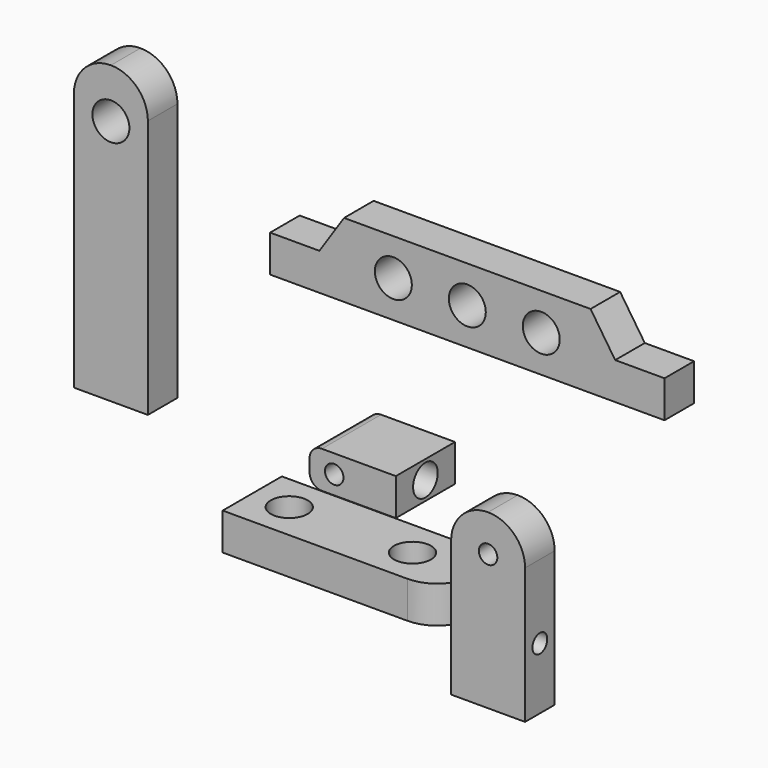
from build123d import *

# Parameters (mm, degrees)
F0_W      = 44.45
F0_H      = 19.05
F1_DEPTH  = 38.1
F2_R      = 4.7625
F3_DEPTH  = 118.58277
F4_R      = 7.9375
F5_DEPTH  = 12.7
F6_R      = 6.35
F7_W      = 38.1
F7_H      = 88.9
F7_R      = 4.7625
F8_DEPTH  = 19.05
F9_R      = 4.7625
F10_DEPTH = 19.05
F11_R     = 19.04999
F12_W     = 114.3
F12_H     = 19.05
F13_DEPTH = 38.1
F14_R     = 9.525
F15_DEPTH = 43.37852
F16_R     = 19.04999
F17_R     = 9.525
F18_DEPTH = 19.05
F19_R     = 9.525
F20_DEPTH = 19.05


# Not quite as in the source:
# - a fillet or chamfer is up to 0.001 mm smaller than in the source, because OpenCascade refuses the exact size


with BuildPart() as f1:
    # F0 (on Front) → F1 (new body)
    with BuildSketch(Plane.XZ):
        with Locations((-4.5246369214, 25.4022409208)):
            Rectangle(F0_W, F0_H)
    extrude(amount=-F1_DEPTH)

    # F2 (on face) → F3 (cut)
    with BuildSketch(Plane.XZ):
        with Locations((-14.0496369214, 25.4022409208)):
            Circle(F2_R)
    extrude(amount=-F3_DEPTH, mode=Mode.SUBTRACT)

    # F4 (on face) → F5 (cut)
    with BuildSketch(Plane.YZ.offset(17.7003630786)):
        with Locations((19.05, 25.4022409208)):
            Circle(F4_R)
    extrude(amount=-F5_DEPTH, mode=Mode.SUBTRACT)

    # F6
    f6_edges = [f1.edges().sort_by_distance(p)[0] for p in [
        (-26.749637, 19.05, 34.927241),
        (-26.749637, 19.05, 15.877241),
    ]]
    fillet(f6_edges, radius=F6_R)


with BuildPart() as f8:
    # F7 (on Front) → F8 (new body)
    with BuildSketch(Plane.XZ):
        with Locations((65.2318205684, -10.4596508645)):
            Rectangle(F7_W, F7_H)
        with Locations((65.2318205684, 14.9403491355)):
            Circle(F7_R, mode=Mode.SUBTRACT)
    extrude(amount=-F8_DEPTH)

    # F9 (on face) → F10 (cut)
    with BuildSketch(Plane.YZ.offset(84.2818205684)):
        with Locations((9.525, -23.1596508645)):
            Circle(F9_R)
    extrude(amount=-F10_DEPTH, mode=Mode.SUBTRACT)

    # F11 (radius 19.05 in the source; OpenCascade refuses exactly that, so slightly less here)
    f11_edges = [f8.edges().sort_by_distance(p)[0] for p in [
        (84.281821, 9.525, 33.990349),
        (46.181821, 9.525, 33.990349),
    ]]
    fillet(f11_edges, radius=F11_R)


with BuildPart() as f13:
    # F12 (on Front) → F13 (new body)
    with BuildSketch(Plane.XZ):
        with Locations((-14.3527926165, -19.2319881171)):
            Rectangle(F12_W, F12_H)
    extrude(amount=-F13_DEPTH)

    # F14 (on face) → F15 (cut)
    with BuildSketch(Plane.XY.offset(-9.7069881171)):
        with Locations((-52.4527926165, 19.05)):
            Circle(F14_R)
        with Locations((11.0472073835, 19.05)):
            Circle(F14_R)
    extrude(amount=-F15_DEPTH, mode=Mode.SUBTRACT)

    # F16 (radius 19.05 in the source; OpenCascade refuses exactly that, so slightly less here)
    f16_edges = [f13.edges().sort_by_distance(p)[0] for p in [
        (42.797207, 38.1, -19.231988),
        (42.797207, 0, -19.231988),
    ]]
    fillet(f16_edges, radius=F16_R)


with BuildPart() as f18:
    # F17 (on Front) → F18 (new body)
    with BuildSketch(Plane.XZ):
        with BuildLine():
            Line((-148.1536233306, 154.4727383056), (-148.1536233306, 21.1227383056))
            Line((-148.1536233306, 21.1227383056), (-110.0536233306, 21.1227383056))
            Line((-110.0536233306, 21.1227383056), (-110.0536233306, 154.4727383056))
            ThreePointArc((-110.0536233306, 154.4727383056), (-115.633239149, 167.9431224872), (-129.1036233306, 173.5227383056))
            ThreePointArc((-129.1036233306, 173.5227383056), (-142.5740075122, 167.9431224872), (-148.1536233306, 154.4727383056))
        make_face()
        with Locations((-129.1036233306, 148.1227383056)):
            Circle(F17_R, mode=Mode.SUBTRACT)
    extrude(amount=-F18_DEPTH)


with BuildPart() as f20:
    # F19 (on Front) → F20 (new body)
    with BuildSketch(Plane.XZ):
        Polygon((118.0211378485, 143.3568834615), (-8.9788621515, 143.3568834615), (-21.6788621515, 124.3068834615), (-47.0788621515, 124.3068834615), (-47.0788621515, 105.2568834615), (156.1211378485, 105.2568834615), (156.1211378485, 124.3068834615), (130.7211378485, 124.3068834615), align=None)
        with Locations((16.4211378485, 124.3068834615)):
            Circle(F19_R, mode=Mode.SUBTRACT)
        with Locations((54.5211378485, 124.3068834615)):
            Circle(F19_R, mode=Mode.SUBTRACT)
        with Locations((92.6211378485, 124.3068834615)):
            Circle(F19_R, mode=Mode.SUBTRACT)
    extrude(amount=-F20_DEPTH)


solid = Compound([f1.part, f8.part, f13.part, f18.part, f20.part])
